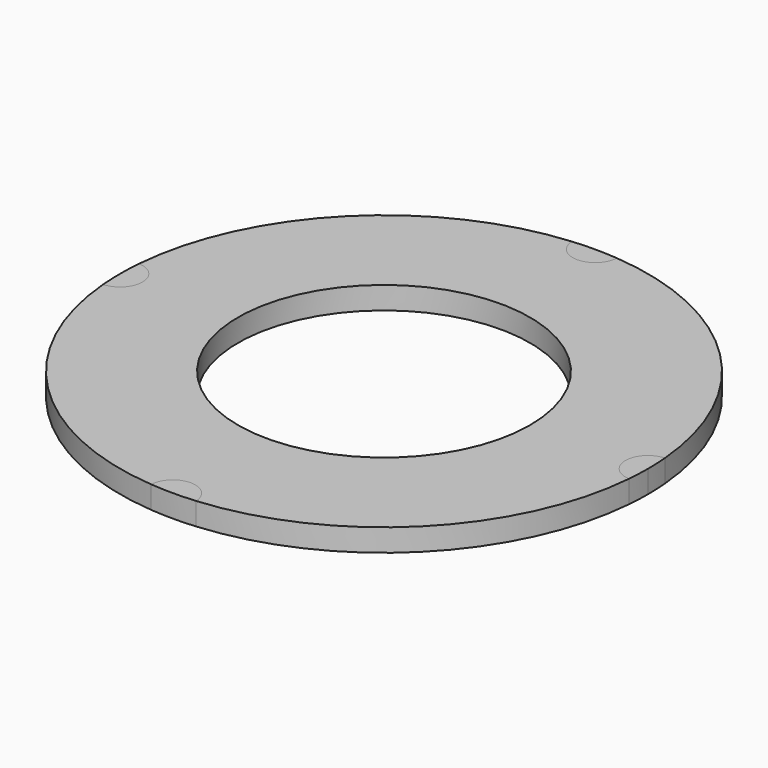
from build123d import *

# Parameters (mm, degrees)
F0_R     = 13
F1_DEPTH = 2
F2_DEPTH = 2


# Not quite as in the source:
# - a feature names something its author has since deleted; it is built from what else it names


with BuildPart() as f1:
    # F0 (on Top) → F1 (new body)
    with BuildSketch(Plane.XY):
        with BuildLine():
            ThreePointArc((21.5, 0), (22.0560102552, 1.383796812), (23.414893617, 1.9981884054))
            ThreePointArc((23.414893617, 1.9981884054), (16.6170093579, 16.6170093579), (1.9981884054, 23.414893617))
            ThreePointArc((1.9981884054, 23.414893617), (1.3837968027, 22.0560102463), (-2.58e-08, 21.5))
            ThreePointArc((-2.58e-08, 21.5), (15.2027957864, 15.2027958046), (21.5, 0))
        make_face()
        with BuildLine():
            ThreePointArc((-2.58e-08, 21.5), (1.3837968027, 22.0560102463), (1.9981884054, 23.414893617))
            ThreePointArc((1.9981884054, 23.414893617), (0, 23.5), (-1.9981884054, 23.414893617))
            ThreePointArc((-1.9981884054, 23.414893617), (-1.3837968214, 22.0560102642), (-2.58e-08, 21.5))
        make_face()
        with BuildLine():
            ThreePointArc((-2.58e-08, 21.5), (-1.3837968214, 22.0560102642), (-1.9981884054, 23.414893617))
            ThreePointArc((-1.9981884054, 23.414893617), (-16.6170093579, 16.6170093579), (-23.414893617, 1.9981884054))
            ThreePointArc((-23.414893617, 1.9981884054), (-22.0560102552, 1.383796812), (-21.5, 0))
            ThreePointArc((-21.5, 0), (-15.2027958046, 15.2027957864), (-2.58e-08, 21.5))
        make_face()
        with BuildLine():
            ThreePointArc((-21.5, 0), (-22.0560102552, 1.383796812), (-23.414893617, 1.9981884054))
            ThreePointArc((-23.414893617, 1.9981884054), (-23.5, 0), (-23.414893617, -1.9981884054))
            ThreePointArc((-23.414893617, -1.9981884054), (-22.0560102552, -1.383796812), (-21.5, 0))
        make_face()
        with BuildLine():
            ThreePointArc((-1.9981884054, -23.414893617), (-1.3837968124, -22.0560102556), (-1.1e-09, -21.5))
            ThreePointArc((-1.1e-09, -21.5), (-15.2027957959, -15.2027957951), (-21.5, 0))
            ThreePointArc((-21.5, 0), (-22.0560102552, -1.383796812), (-23.414893617, -1.9981884054))
            ThreePointArc((-23.414893617, -1.9981884054), (-16.6170093579, -16.6170093579), (-1.9981884054, -23.414893617))
        make_face()
        with BuildLine():
            ThreePointArc((-1.9981884054, -23.414893617), (0, -23.5), (1.9981884054, -23.414893617))
            ThreePointArc((1.9981884054, -23.414893617), (1.3837968117, -22.0560102549), (-1.1e-09, -21.5))
            ThreePointArc((-1.1e-09, -21.5), (-1.3837968124, -22.0560102556), (-1.9981884054, -23.414893617))
        make_face()
        with BuildLine():
            ThreePointArc((1.9981884054, -23.414893617), (16.6170093579, -16.6170093579), (23.414893617, -1.9981884054))
            ThreePointArc((23.414893617, -1.9981884054), (22.0560102552, -1.383796812), (21.5, 0))
            ThreePointArc((21.5, 0), (15.2027957951, -15.2027957959), (-1.1e-09, -21.5))
            ThreePointArc((-1.1e-09, -21.5), (1.3837968117, -22.0560102549), (1.9981884054, -23.414893617))
        make_face()
        with BuildLine():
            ThreePointArc((23.414893617, -1.9981884054), (23.4787137637, -1), (23.5, 0))
            ThreePointArc((23.5, 0), (23.4787137637, 1), (23.414893617, 1.9981884054))
            ThreePointArc((23.414893617, 1.9981884054), (22.0560102552, 1.383796812), (21.5, 0))
            ThreePointArc((21.5, 0), (22.0560102552, -1.383796812), (23.414893617, -1.9981884054))
        make_face()
        with BuildLine():
            ThreePointArc((-1.1e-09, -21.5), (15.2027957951, -15.2027957959), (21.5, 0))
            ThreePointArc((21.5, 0), (15.2027957864, 15.2027958046), (-2.58e-08, 21.5))
            ThreePointArc((-2.58e-08, 21.5), (-15.2027958046, 15.2027957864), (-21.5, 0))
            ThreePointArc((-21.5, 0), (-15.2027957959, -15.2027957951), (-1.1e-09, -21.5))
        make_face()
        Circle(F0_R, mode=Mode.SUBTRACT)
    extrude(amount=F1_DEPTH)


with BuildPart() as f2:
    # F0 (on Top) → F2 (new body)
    with BuildSketch(Plane.XY):
        with BuildLine():
            ThreePointArc((-1.1e-09, -21.5), (15.2027957951, -15.2027957959), (21.5, 0))
            ThreePointArc((21.5, 0), (15.2027957864, 15.2027958046), (-2.58e-08, 21.5))
            ThreePointArc((-2.58e-08, 21.5), (-15.2027958046, 15.2027957864), (-21.5, 0))
            ThreePointArc((-21.5, 0), (-15.2027957959, -15.2027957951), (-1.1e-09, -21.5))
        make_face()
        Circle(F0_R, mode=Mode.SUBTRACT)
        with BuildLine():
            ThreePointArc((-1.9981884054, -23.414893617), (-1.3837968124, -22.0560102556), (-1.1e-09, -21.5))
            ThreePointArc((-1.1e-09, -21.5), (-15.2027957959, -15.2027957951), (-21.5, 0))
            ThreePointArc((-21.5, 0), (-22.0560102552, -1.383796812), (-23.414893617, -1.9981884054))
            ThreePointArc((-23.414893617, -1.9981884054), (-16.6170093579, -16.6170093579), (-1.9981884054, -23.414893617))
        make_face()
        with BuildLine():
            ThreePointArc((-2.58e-08, 21.5), (-1.3837968214, 22.0560102642), (-1.9981884054, 23.414893617))
            ThreePointArc((-1.9981884054, 23.414893617), (-16.6170093579, 16.6170093579), (-23.414893617, 1.9981884054))
            ThreePointArc((-23.414893617, 1.9981884054), (-22.0560102552, 1.383796812), (-21.5, 0))
            ThreePointArc((-21.5, 0), (-15.2027958046, 15.2027957864), (-2.58e-08, 21.5))
        make_face()
        with BuildLine():
            ThreePointArc((1.9981884054, -23.414893617), (16.6170093579, -16.6170093579), (23.414893617, -1.9981884054))
            ThreePointArc((23.414893617, -1.9981884054), (22.0560102552, -1.383796812), (21.5, 0))
            ThreePointArc((21.5, 0), (15.2027957951, -15.2027957959), (-1.1e-09, -21.5))
            ThreePointArc((-1.1e-09, -21.5), (1.3837968117, -22.0560102549), (1.9981884054, -23.414893617))
        make_face()
        with BuildLine():
            ThreePointArc((21.5, 0), (22.0560102552, 1.383796812), (23.414893617, 1.9981884054))
            ThreePointArc((23.414893617, 1.9981884054), (16.6170093579, 16.6170093579), (1.9981884054, 23.414893617))
            ThreePointArc((1.9981884054, 23.414893617), (1.3837968027, 22.0560102463), (-2.58e-08, 21.5))
            ThreePointArc((-2.58e-08, 21.5), (15.2027957864, 15.2027958046), (21.5, 0))
        make_face()
    extrude(amount=F2_DEPTH)


solid = Compound([f1.part, f2.part])
